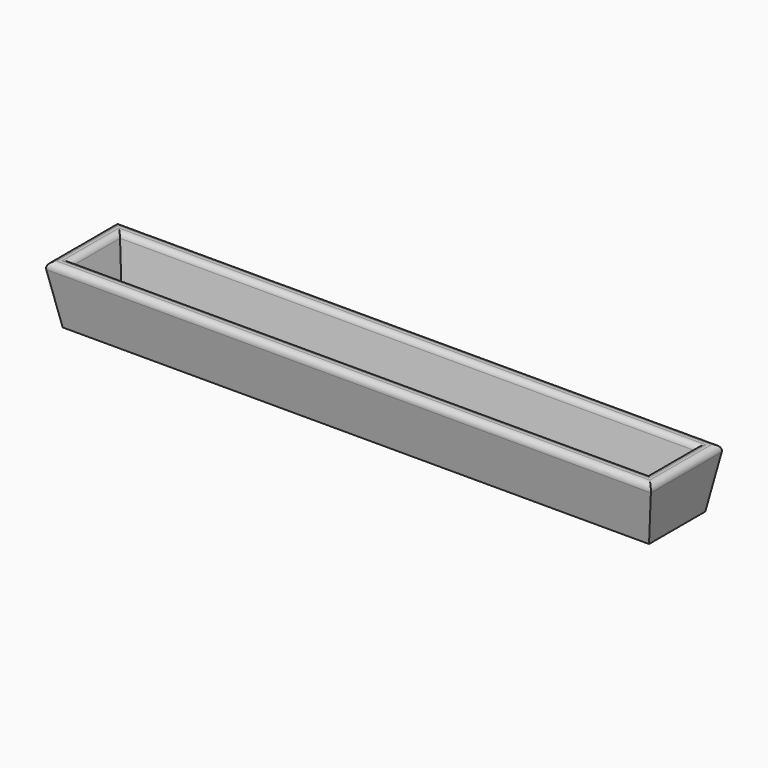
from build123d import *

# Parameters (mm, degrees)
F0_W     = 100
F0_H     = 12
F1_DEPTH = 10
F1_TAPER = -10
F2_T     = -2.5
F3_R     = 1


with BuildPart() as f1:
    # F0 (on Top) → F1 (new body)
    with BuildSketch(Plane.XY):
        with Locations((-1.4750659466, -34.9569652333)):
            Rectangle(F0_W, F0_H)
    extrude(amount=F1_DEPTH, taper=F1_TAPER)

    # F2
    f2_openings = [f1.faces().sort_by_distance(p)[0] for p in [
        (-1.475066, -34.956965, 10),
    ]]
    offset(amount=F2_T, openings=f2_openings)

    # F3
    f3_edges = [f1.edges().sort_by_distance(p)[0] for p in [
        (-1.475066, -42.720235, 10),
        (-53.238336, -34.956965, 10),
        (-1.475066, -27.193695, 10),
        (50.288204, -34.956965, 10),
        (-1.475066, -29.732262, 10),
        (47.749637, -34.956965, 10),
        (-1.475066, -40.181669, 10),
        (-50.699769, -34.956965, 10),
    ]]
    fillet(f3_edges, radius=F3_R)


solid = f1.part
